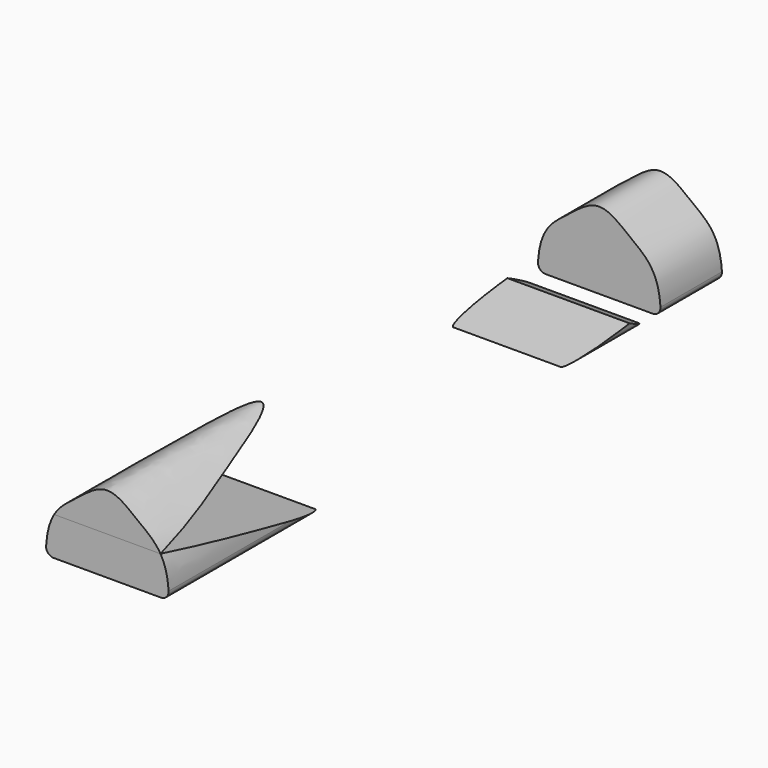
from build123d import *

# Parameters (mm, degrees)
F2_DEPTH = 9000
F0_W     = 8000
F0_H     = 2000
F3_DEPTH = 2500


with BuildPart() as f2:
    # F1 (on Front) → F2 (new body, symmetric)
    with BuildSketch(Plane.XZ):
        with BuildLine():
            ThreePointArc((-1593.8242572385, -787.8322373844), (-1539.854532805, -937.0519016228), (-1394.1947364933, -1000))
            Line((-1394.1947364933, -1000), (1394.1947364933, -1000))
            ThreePointArc((1394.1947364933, -1000), (1539.854532805, -937.0519016228), (1593.8242572385, -787.8322373844))
            add(Edge.make_bspline(
                [(-1593.8242572385, -787.8322373844), (-1543.6100586497, 36.0033941567), (-911.3761259503, 443.0558884844), (0, 1250.1154223925), (911.3761259503, 443.0558884844), (1543.6100586497, 36.0033941567), (1593.8242572385, -787.8322373844)],
                knots=[0.0213435754, 0.0213435754, 0.0213435754, 0.0213435754, 0.2850424282, 0.5, 0.7149575718, 0.9786564246, 0.9786564246, 0.9786564246, 0.9786564246], degree=3))
        make_face()
    extrude(amount=F2_DEPTH, both=True)

    # F0 (on Right) → F3 (cut, symmetric)
    with BuildSketch(Plane.YZ):
        Rectangle(F0_W, F0_H)
        Polygon((-4000, -1000), (-4000, 1000), (-9000, 0), align=None)
        Polygon((6000, 1000), (4000, 1000), (4000, -1000), (6000, -750), align=None)
        Polygon((7000, 1000), (6000, 1000), (6000, -750), (7000, -1250), align=None)
    extrude(amount=F3_DEPTH, both=True, mode=Mode.SUBTRACT)


solid = f2.part
